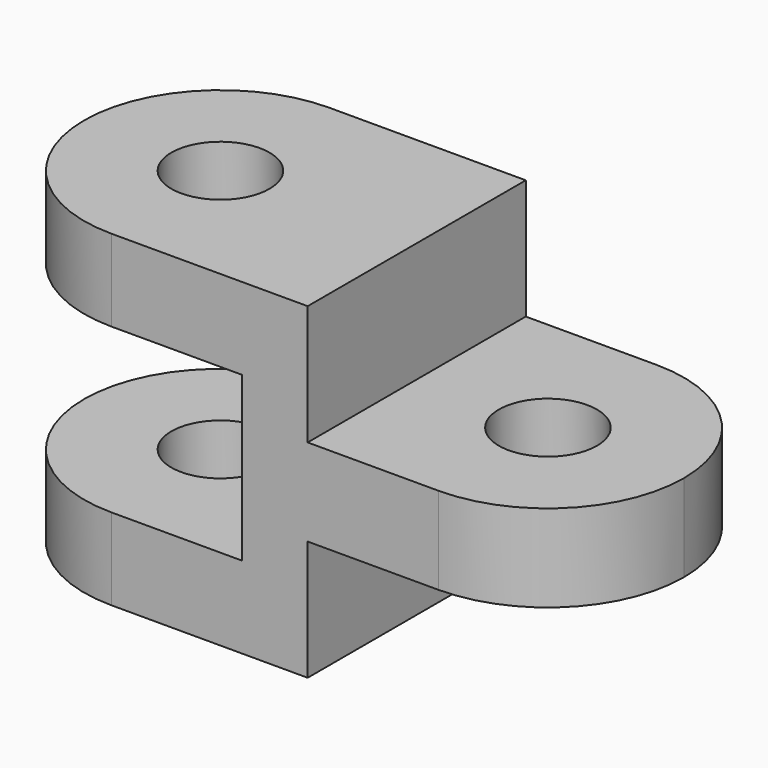
from build123d import *

# Parameters (mm, degrees)
F1_DEPTH = 50
F2_R     = 24.99999
F3_R     = 9
F5_DEPTH = 60.001
F6_R     = 9
F7_DEPTH = 25.4


# Not quite as in the source:
# - a fillet or chamfer is up to 0.001 mm smaller than in the source, because OpenCascade refuses the exact size


with BuildPart() as f1:
    # F0 (on Front) → F1 (new body)
    with BuildSketch(Plane.XZ):
        Polygon((-110, 0), (-49, 0), (-49, 22), (0, 22), (0, 38), (-49, 38), (-49, 60), (-110, 60), (-110, 45), (-61, 45), (-61, 15), (-110, 15), align=None)
    extrude(amount=F1_DEPTH)

    # F2 (radius 25 in the source; OpenCascade refuses exactly that, so slightly less here)
    f2_edges = [f1.edges().sort_by_distance(p)[0] for p in [
        (-110, -50, 52.5),
        (-110, -50, 7.5),
        (-110, 0, 52.5),
        (-110, 0, 7.5),
        (0, -50, 30),
        (0, 0, 30),
    ]]
    fillet(f2_edges, radius=F2_R)

    # F3 (on face) → F5 (cut, through all)
    with BuildSketch(Plane(origin=(0, 0, 0), x_dir=(1, 0, 0), z_dir=(0, 0, -1))):
        with Locations((-85, 25)):
            Circle(F3_R)
    extrude(amount=-F5_DEPTH, mode=Mode.SUBTRACT)

    # F6 (on face) → F7 (cut)
    with BuildSketch(Plane(origin=(0, 0, 22), x_dir=(1, 0, 0), z_dir=(0, 0, -1))):
        with Locations((-25, 24.9226680556)):
            Circle(F6_R)
    extrude(amount=-F7_DEPTH, mode=Mode.SUBTRACT)


solid = f1.part
